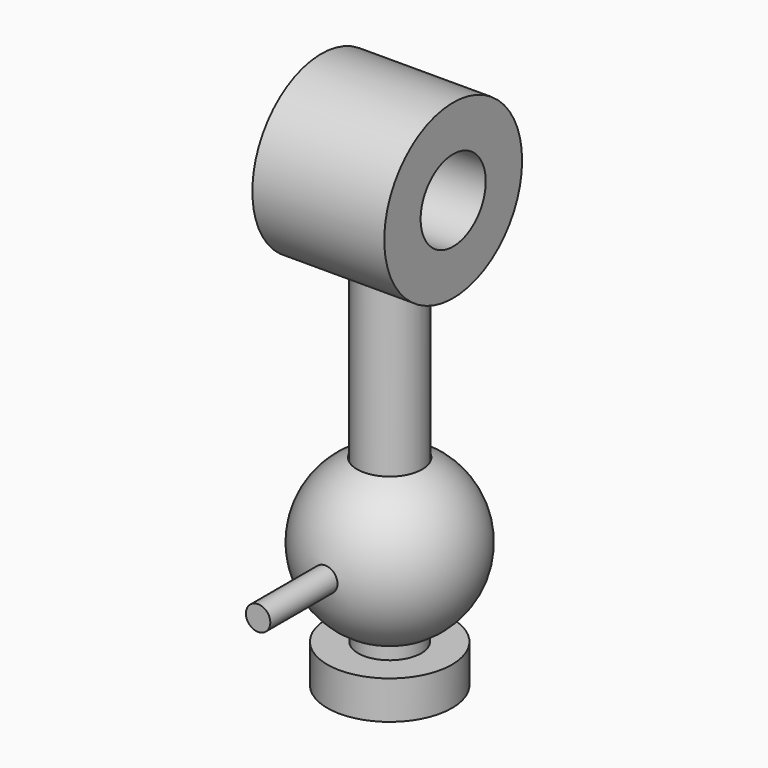
from build123d import *

# Parameters (mm, degrees)
F0_R      = 1.5
F1_DEPTH  = 20.2
F4_R      = 4
F5_DEPTH  = 45.1
F8_DEPTH  = 25
F12_R     = 3.9
F13_DEPTH = 48
F15_R     = 3.875
F16_DEPTH = 32
F18_R     = 7.6531254966
F19_DEPTH = 4.7
F20_R     = 10.5817135641
F21_DEPTH = 7.8
F22_DEPTH = 16.2
F23_R     = 5
F24_DEPTH = 25


# Not quite as in the source:
# - a feature of the source that left no trace in its solid (it failed there, or was rolled back) is left out


with BuildPart() as f1:
    # F0 (on Front) → F1 (new body)
    with BuildSketch(Plane.XZ):
        with Locations((0, 8.262563113)):
            Circle(F0_R)
    extrude(amount=F1_DEPTH)

    # F2 (on Front) → F3 (revolve)
    with BuildSketch(Plane.XZ):
        with BuildLine():
            Line((0, -1.737436887), (0, 18.262563113))
            ThreePointArc((0, 18.262563113), (-10, 8.262563113), (0, -1.737436887))
        make_face()
    revolve(axis=Axis((0, 0, 8.262563113), (0, 0, -1)))

    # F4 (on Top) → F5 (cut)
    with BuildSketch(Plane.XY):
        Circle(F4_R)
    extrude(amount=F5_DEPTH, mode=Mode.SUBTRACT)

    # F4 (on Top) → F8 (cut)
    with BuildSketch(Plane.XY):
        Circle(F4_R)
    extrude(amount=-F8_DEPTH, mode=Mode.SUBTRACT)


with BuildPart() as f13:
    # F12 (on Top) → F13 (new body)
    with BuildSketch(Plane.XY):
        Circle(F12_R)
    extrude(amount=F13_DEPTH)

    # F15 (on offset) → F16 (join)
    with BuildSketch(Plane.XY.offset(25)):
        Circle(F15_R)
    extrude(amount=-F16_DEPTH)

    # F18 (on offset) → F19 (join)
    with BuildSketch(Plane.XY.offset(-2.5)):
        Circle(F18_R)
    extrude(amount=-F19_DEPTH)

    # F20 (on Right) → F21 (join)
    with BuildSketch(Plane.YZ):
        with Locations((0, 47.7548092604)):
            Circle(F20_R)
    extrude(amount=F21_DEPTH)

    # F22 (add): a face of the model
    f22_faces = [f13.faces().sort_by_distance(p)[0] for p in [
        (7.8, 0, 47.7548092604),
    ]]
    extrude(f22_faces, amount=-F22_DEPTH)

    # F23 (on face) → F24 (cut)
    with BuildSketch(Plane(origin=(-8.4, 0, 0), x_dir=(0, -1, 0), z_dir=(-1, 0, 0))):
        with Locations((0, 47.7548092604)):
            Circle(F23_R)
    extrude(amount=-F24_DEPTH, mode=Mode.SUBTRACT)


solid = Compound([f1.part, f13.part])
